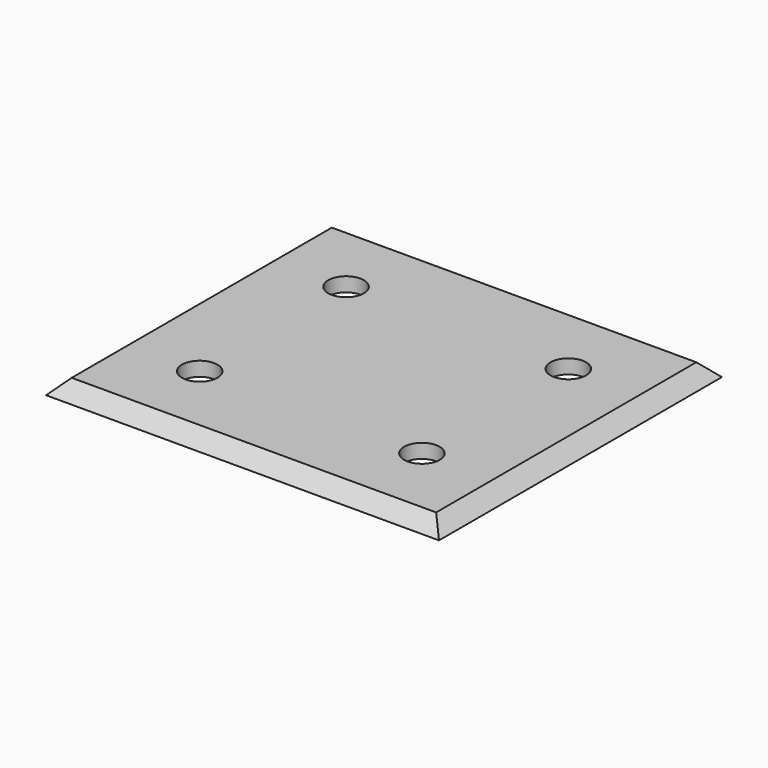
from build123d import *

# Parameters (mm, degrees)
F0_W        = 61.2471848726
F0_H        = 55.7258352637
F1_DEPTH    = 2
F4_D        = 5
F5_T1_DEPTH = 81.4426651434
F5_T3_DEPTH = 86.9640147523


# Not quite as in the source:
# - a fillet or chamfer that OpenCascade refuses, or shapes differently, is made with other operations: its cross-section is extruded or revolved along the edge and cut away or added


with BuildPart() as f1:
    # F0 (on Top) → F1 (new body)
    with BuildSketch(Plane.XY):
        with Locations((30.6235924363, 27.8629176319)):
            Rectangle(F0_W, F0_H)
    extrude(amount=F1_DEPTH)

    # F4 (through all)
    with Locations(Plane(origin=(0, 0, 0), x_dir=(1, 0, 0), z_dir=(0, 0, -1))):
        with Locations((15, -40.7258352637), (46.2471848726, -40.7258352637), (15, -15), (46.2471848726, -15)):
            Hole(F4_D / 2)

    # F5: chamfer of 5 on 4 edges, made by hand

    # F5_s2 → F5_t1 (cut)
    with BuildSketch(Plane.XZ.offset(-68.5842502036)):
        Polygon((0, -3), (5, 2), (0, 2), align=None)
        Polygon((56.2471848726, 2), (61.2471848726, -3), (61.2471848726, 2), align=None)
    extrude(amount=F5_T1_DEPTH, mode=Mode.SUBTRACT)

    # F5_s4 → F5_t3 (cut)
    with BuildSketch(Plane.YZ.offset(-12.8584149398)):
        Polygon((55.7258352637, -3), (50.7258352637, 2), (55.7258352637, 2), align=None)
        Polygon((0, -3), (5, 2), (0, 2), align=None)
    extrude(amount=F5_T3_DEPTH, mode=Mode.SUBTRACT)


solid = f1.part
